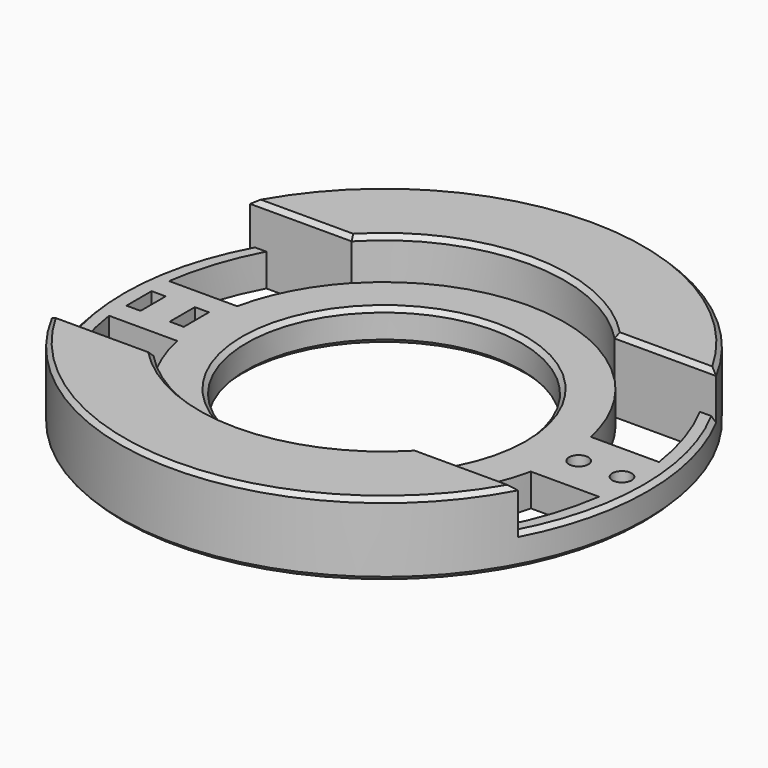
from build123d import *

# Parameters (mm, degrees)
F0_R      = 61
F0_W      = 3.2512
F0_H      = 7.2644
F0_R_2    = 2.2352
F1_DEPTH  = 12
F2_R      = 41.785
F2_R_2    = 31.785
F3_DEPTH  = 2.5
F6_W      = 128.4000128508
F6_H      = 40
F7_DEPTH  = 9.5
F10_D     = 83.5
F11_R     = 41.785
F11_R_2   = 31.785
F12_DEPTH = 2.5
F14_DEPTH = 2.501
F15_W     = 126.7949044704
F15_H     = 57.2644
F16_DEPTH = 9.5
F18_ANGLE = 180
F19_DEPTH = 5
F20_SIZE  = 1


with BuildPart() as f1:
    # F0 (on Top) → F1 (new body)
    with BuildSketch(Plane.XY):
        Circle(F0_R)
        with Locations((-55, 0)):
            Rectangle(F0_W, F0_H, mode=Mode.SUBTRACT)
        with Locations((-45, 0)):
            Rectangle(F0_W, F0_H, mode=Mode.SUBTRACT)
        with Locations((45, 0)):
            Circle(F0_R_2, mode=Mode.SUBTRACT)
        with Locations((55, 0)):
            Circle(F0_R_2, mode=Mode.SUBTRACT)
    extrude(amount=F1_DEPTH)

    # F2 (on face) → F3 (join)
    with BuildSketch(Plane.XY.offset(12)):
        Circle(F2_R)
        Circle(F2_R_2, mode=Mode.SUBTRACT)
    extrude(amount=-F3_DEPTH)

    # F6 (on face) → F7 (cut)
    with BuildSketch(Plane(origin=(0, 0, 0), x_dir=(1, 0, 0), z_dir=(0, 0, -1))):
        Rectangle(F6_W, F6_H)
    extrude(amount=-F7_DEPTH, mode=Mode.SUBTRACT)

    # F10 (through all)
    with Locations(Plane(origin=(0, 0, -150), x_dir=(1, 0, 0), z_dir=(0, 0, -1))):
        with Locations((0, 0)):
            Hole(F10_D / 2)

    # F11 (on face) → F12 (join, through all)
    with BuildSketch(Plane.XY.offset(12)):
        Circle(F11_R)
        Circle(F11_R_2, mode=Mode.SUBTRACT)
    extrude(amount=-F12_DEPTH)

    # F13 (on face) → F14 (cut, through all)
    with BuildSketch(Plane(origin=(0, 0, 9.5), x_dir=(1, 0, 0), z_dir=(0, 0, -1))):
        with BuildLine():
            ThreePointArc((-50.108761934, 28.6322), (-54.2322806707, 18.9365058544), (-56.6256, 8.6758082989))
            Line((-56.6256, 8.6758082989), (-40.8744, 8.6758082989))
            ThreePointArc((-40.8744, 8.6758082989), (-37.0237762252, 19.3707568005), (-30.4332605575, 28.6322))
            Line((-30.4332605575, 28.6322), (-50.108761934, 28.6322))
        make_face()
        with BuildLine():
            Line((50.108761934, 28.6322), (30.4332605575, 28.6322))
            ThreePointArc((30.4332605575, 28.6322), (37.0237762252, 19.3707568005), (40.8744, 8.6758082989))
            Line((40.8744, 8.6758082989), (56.6256, 8.6758082989))
            ThreePointArc((56.6256, 8.6758082989), (54.2322806707, 18.9365058544), (50.108761934, 28.6322))
        make_face()
        with BuildLine():
            Line((-40.8744, -8.6758082989), (-56.6256, -8.6758082989))
            ThreePointArc((-56.6256, -8.6758082989), (-54.2322806707, -18.9365058544), (-50.108761934, -28.6322))
            Line((-50.108761934, -28.6322), (-30.4332605575, -28.6322))
            ThreePointArc((-30.4332605575, -28.6322), (-37.0237762252, -19.3707568005), (-40.8744, -8.6758082989))
        make_face()
        with BuildLine():
            ThreePointArc((40.8744, -8.6758082989), (37.0237762252, -19.3707568005), (30.4332605575, -28.6322))
            Line((30.4332605575, -28.6322), (50.108761934, -28.6322))
            ThreePointArc((50.108761934, -28.6322), (54.2322806707, -18.9365058544), (56.6256, -8.6758082989))
            Line((56.6256, -8.6758082989), (40.8744, -8.6758082989))
        make_face()
    extrude(amount=-F14_DEPTH, mode=Mode.SUBTRACT)

    # F15 (on face) → F16 (cut, through all)
    with BuildSketch(Plane(origin=(0, 0, 0), x_dir=(1, 0, 0), z_dir=(0, 0, -1))):
        Rectangle(F15_W, F15_H)
    extrude(amount=-F16_DEPTH, mode=Mode.SUBTRACT)


with BuildPart() as f1_1:
    # F18: moved
    add(f1.part.rotate(Axis((-38.5658666492, 0, 0), (-1, 0, 0)), F18_ANGLE))

    # F19 (add): a face of the model
    f19_faces = [f1_1.faces().sort_by_distance(p)[0] for p in [
        (-59.2746594539, 0, -12),
    ]]
    extrude(f19_faces, amount=F19_DEPTH)

    # F20
    f20_edges = [f1_1.edges().sort_by_distance(p)[0] for p in [
        (-31.785, 0, -9.5),
        (42.123975, -28.6322, 0),
        (-42.123975, -28.6322, 0),
        (0, -61, 0),
        (-42.123975, 28.6322, 0),
        (42.123975, 28.6322, 0),
        (0, 61, 0),
        (-31.785, 0, -17),
        (-61, 0, -17),
        (59.188802, -14.754178, -9.5),
        (59.188802, 14.754178, -9.5),
        (-61, 0, -9.5),
        (0, -41.75, 0),
        (0, 41.75, 0),
    ]]
    chamfer(f20_edges, length=F20_SIZE)


solid = f1_1.part
